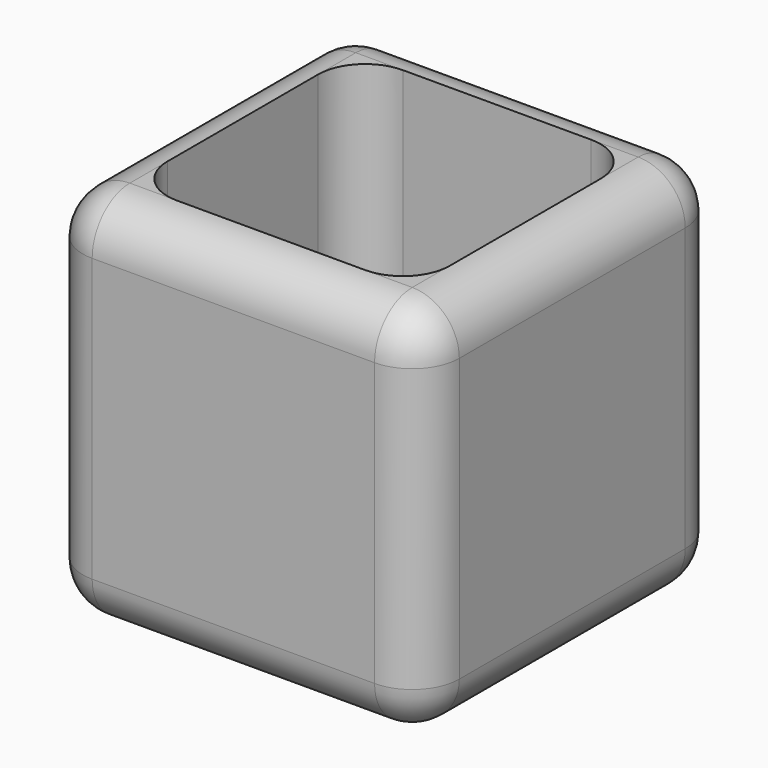
from build123d import *

# Parameters (mm, degrees)
F0_W      = 203.2
F0_H      = 203.2
F1_DEPTH  = 203.2
F2_R      = 25.4
F3_W      = 50.8
F3_H      = 50.8
F4_DEPTH  = 12.7
F5_W      = 50.8
F5_H      = 50.8
F6_DEPTH  = 12.7
F12_DEPTH = 177.8


# Not quite as in the source:
# - a feature of the source that left no trace in its solid (it failed there, or was rolled back) is left out


with BuildPart() as f1:
    # F0 (on Top) → F1 (new body)
    with BuildSketch(Plane.XY):
        Rectangle(F0_W, F0_H)
    extrude(amount=F1_DEPTH)

    # F2
    f2_edges = [f1.edges().sort_by_distance(p)[0] for p in [
        (0, 101.6, 203.2),
        (-101.6, 0, 203.2),
        (0, -101.6, 203.2),
        (101.6, 0, 203.2),
        (-101.6, -101.6, 101.6),
        (101.6, -101.6, 101.6),
        (0, -101.6, 0),
        (-101.6, 101.6, 101.6),
        (-101.6, 0, 0),
        (101.6, 101.6, 101.6),
        (0, 101.6, 0),
        (101.6, 0, 0),
    ]]
    fillet(f2_edges, radius=F2_R)

    # F3 (on face) → F4 (cut)
    with BuildSketch(Plane.XY.offset(203.2)):
        with BuildLine():
            Line((50.8, 76.2), (-50.8, 76.2))
            ThreePointArc((-50.8, 76.2), (-68.7605122421, 68.7605122421), (-76.2, 50.8))
            Line((-76.2, 50.8), (-76.2, -50.8))
            ThreePointArc((-76.2, -50.8), (-68.7605122421, -68.7605122421), (-50.8, -76.2))
            Line((-50.8, -76.2), (50.8, -76.2))
            ThreePointArc((50.8, -76.2), (68.7605122421, -68.7605122421), (76.2, -50.8))
            Line((76.2, -50.8), (76.2, 50.8))
            ThreePointArc((76.2, 50.8), (68.7605122421, 68.7605122421), (50.8, 76.2))
        make_face()
        Rectangle(F3_W, F3_H, mode=Mode.SUBTRACT)
    extrude(amount=-F4_DEPTH, mode=Mode.SUBTRACT)

    # F5 (on face) → F6 (cut)
    with BuildSketch(Plane.XY.offset(203.2)):
        with BuildLine():
            Line((-25.4, 25.4), (25.4, 25.4))
            ThreePointArc((25.4, 25.4), (0, 35.9210244843), (-25.4, 25.4))
        make_face()
        with BuildLine():
            Line((-25.4, -25.4), (-25.4, 25.4))
            ThreePointArc((-25.4, 25.4), (-35.9210244843, 0), (-25.4, -25.4))
        make_face()
        with BuildLine():
            ThreePointArc((-25.4, -25.4), (0, -35.9210244843), (25.4, -25.4))
            Line((25.4, -25.4), (-25.4, -25.4))
        make_face()
        Rectangle(F5_W, F5_H)
        with BuildLine():
            ThreePointArc((25.4, -25.4), (33.1866993079, -13.7463809437), (35.9210244843, 0))
            ThreePointArc((35.9210244843, 0), (33.1866993079, 13.7463809437), (25.4, 25.4))
            Line((25.4, 25.4), (25.4, -25.4))
        make_face()
    extrude(amount=-F6_DEPTH, mode=Mode.SUBTRACT)

    # F11 (on offset) → F12 (cut)
    with BuildSketch(Plane.XY.offset(228.6)):
        with BuildLine():
            Line((50.8, 76.2), (-50.8, 76.2))
            ThreePointArc((-50.8, 76.2), (-68.7605122421, 68.7605122421), (-76.2, 50.8))
            Line((-76.2, 50.8), (-76.2, -50.8))
            ThreePointArc((-76.2, -50.8), (-68.7605122421, -68.7605122421), (-50.8, -76.2))
            Line((-50.8, -76.2), (50.8, -76.2))
            ThreePointArc((50.8, -76.2), (68.7605122421, -68.7605122421), (76.2, -50.8))
            Line((76.2, -50.8), (76.2, 50.8))
            ThreePointArc((76.2, 50.8), (68.7605122421, 68.7605122421), (50.8, 76.2))
        make_face()
    extrude(amount=-F12_DEPTH, mode=Mode.SUBTRACT)


solid = f1.part
